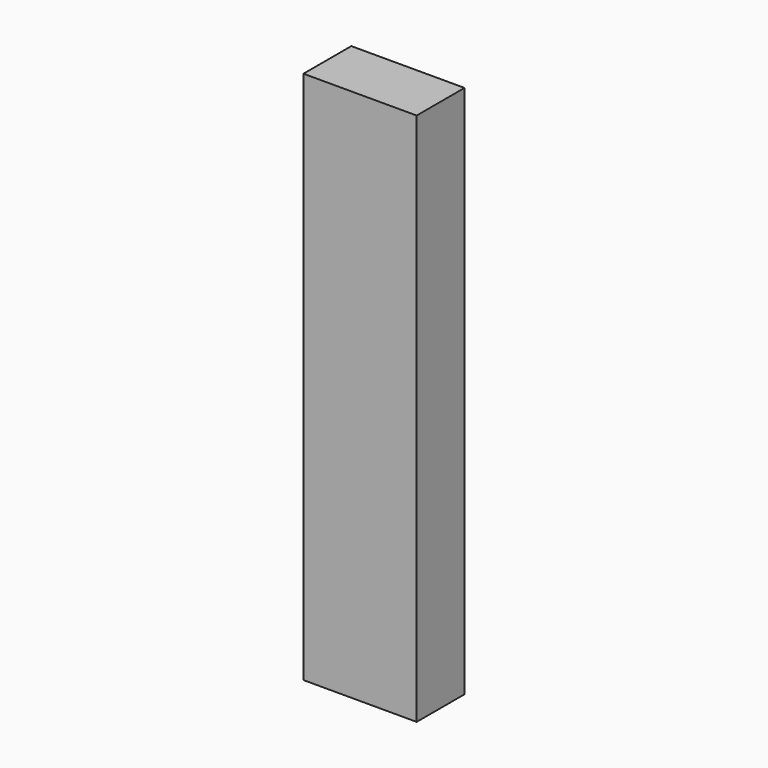
from build123d import *

# Parameters (mm, degrees)
F0_TEXT_SIZE = 62.5
F1_DEPTH     = 5


# Not quite as in the source:
# - Text() gives the source's letters only with a copy of the font that has no kerning and outlines rounded to 1/6400 em; it was checked with that copy


with BuildPart() as f1:
    # F0 (on Front) → F1 (new body)
    with BuildSketch(Plane.XZ):
        with Locations((-49.1197152333, 5.809858499)):
            Text('I', F0_TEXT_SIZE, font='Open Sans', font_style=FontStyle.BOLD, text_align=(TextAlign.LEFT, TextAlign.BOTTOM))
    extrude(amount=F1_DEPTH)


solid = f1.part
